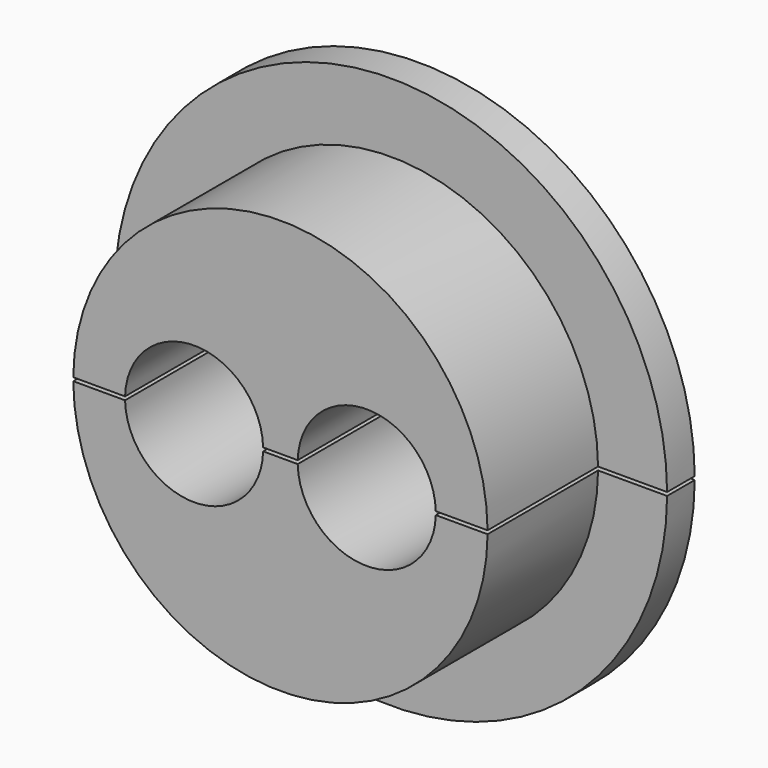
from build123d import *

# Parameters (mm, degrees)
F0_R          = 6
F0_R_2        = 2
F1_DEPTH      = 5
F2_R          = 8
F2_R_2        = 6
F3_DEPTH      = 1
F4_W          = 30
F4_H          = 0.1
F5_DEPTH      = 26
F5_DEPTH_BACK = 5.001


# Not quite as in the source:
# - an extrude ends at something that could not be found from the text; its depth is read off the source's solid


with BuildPart() as f1:
    # F0 (on Front) → F1 (new body)
    with BuildSketch(Plane.XZ):
        Circle(F0_R)
        with Locations((-2.5, 0)):
            Circle(F0_R_2, mode=Mode.SUBTRACT)
        with Locations((2.5, 0)):
            Circle(F0_R_2, mode=Mode.SUBTRACT)
    extrude(amount=F1_DEPTH)

    # F2 (on face) → F3 (join)
    with BuildSketch(Plane(origin=(0, 0, 0), x_dir=(-1, 0, 0), z_dir=(0, 1, 0))):
        Circle(F2_R)
        Circle(F2_R_2, mode=Mode.SUBTRACT)
    extrude(amount=-F3_DEPTH)

    # F4 (on Front) → F5 (cut, two sides)
    with BuildSketch(Plane.XZ) as f5_sk:
        with Locations((0.0164873028, 0)):
            Rectangle(F4_W, F4_H)
    extrude(amount=-F5_DEPTH, mode=Mode.SUBTRACT)
    extrude(f5_sk.sketch, amount=F5_DEPTH_BACK, mode=Mode.SUBTRACT)


solid = f1.part
